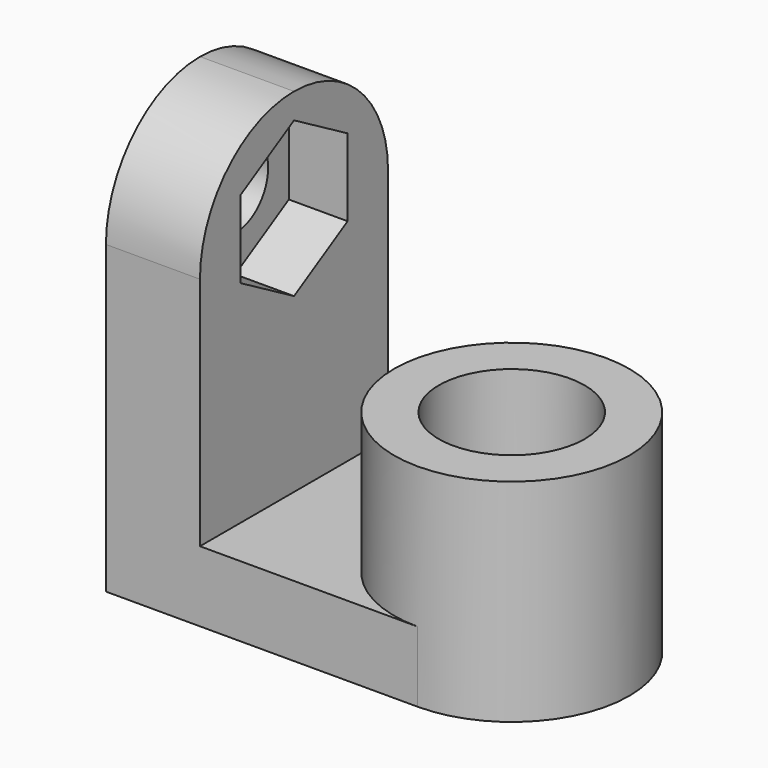
from build123d import *
from build123d import SkipClean  # not in build123d's __all__

# Parameters (mm, degrees)
F0_R      = 3.1
F0_R_2    = 1
F1_DEPTH  = 3
F2_DEPTH  = 6
F3_W      = 4
F3_H      = 10
F4_DEPTH  = 15
F5_R      = 1.75
F6_DEPTH  = 25
F8_DEPTH  = 2.5
F9_R      = 4.99999
F10_W     = 6
F10_H     = 0.4
F11_DEPTH = 25


# Not quite as in the source:
# - a fillet or chamfer is up to 0.001 mm smaller than in the source, because OpenCascade refuses the exact size
# - after a boolean that leaves OpenCascade's solid faulty, fix() repairs it


with BuildPart() as f1:
    # F0 (on Top) → F1 (new body)
    with BuildSketch(Plane.XY):
        with BuildLine():
            ThreePointArc((0, -5), (3.5355339059, -3.5355339059), (5, 0))
            ThreePointArc((5, 0), (3.5355339059, 3.5355339059), (0, 5))
            ThreePointArc((0, 5), (-5, 0), (0, -5))
        make_face()
        Circle(F0_R, mode=Mode.SUBTRACT)
        Circle(F0_R)
        Circle(F0_R_2, mode=Mode.SUBTRACT)
        with BuildLine():
            ThreePointArc((0, -5), (-5, 0), (0, 5))
            Line((0, 5), (-13.260579668, 5))
            Line((-13.260579668, 5), (-13.260579668, -5))
            Line((-13.260579668, -5), (0, -5))
        make_face()
        Circle(F0_R_2)
    extrude(amount=-F1_DEPTH)

    # F0 (on Top) → F2 (join)
    with BuildSketch(Plane.XY):
        with BuildLine():
            ThreePointArc((0, -5), (3.5355339059, -3.5355339059), (5, 0))
            ThreePointArc((5, 0), (3.5355339059, 3.5355339059), (0, 5))
            ThreePointArc((0, 5), (-5, 0), (0, -5))
        make_face()
        Circle(F0_R, mode=Mode.SUBTRACT)
    with SkipClean():  # cleaning this boolean's faces spoils the solid; the shape is the same uncleaned
        extrude(amount=F2_DEPTH)

    # F3 (on face) → F4 (join)
    with BuildSketch(Plane.XY):
        with Locations((-11.260579668, 0)):
            Rectangle(F3_W, F3_H)
    extrude(amount=F4_DEPTH)

    add(f1.part.fix(), mode=Mode.REPLACE)

    # F5 (on face) → F6 (cut)
    with BuildSketch(Plane.YZ.offset(-9.260579668)):
        with Locations((0, 10.6251845136)):
            Circle(F5_R)
    extrude(amount=-F6_DEPTH, mode=Mode.SUBTRACT)

    # F7 (on face) → F8 (cut)
    with BuildSketch(Plane.YZ.offset(-9.260579668)):
        Polygon((0, 7.3342879792), (2.85, 8.9797362464), (2.85, 12.2706327808), (0, 13.916081048), (-2.85, 12.2706327808), (-2.85, 8.9797362464), align=None)
    extrude(amount=-F8_DEPTH, mode=Mode.SUBTRACT)

    # F9 (radius 5 in the source; OpenCascade refuses exactly that, so slightly less here)
    f9_edges = [f1.edges().sort_by_distance(p)[0] for p in [
        (-11.26058, -5, 15),
        (-11.26058, 5, 15),
    ]]
    fillet(f9_edges, radius=F9_R)

    # F10 (on face) → F11 (cut)
    with BuildSketch(Plane.XY):
        Rectangle(F10_W, F10_H)
    extrude(amount=-F11_DEPTH, mode=Mode.SUBTRACT)


solid = f1.part
